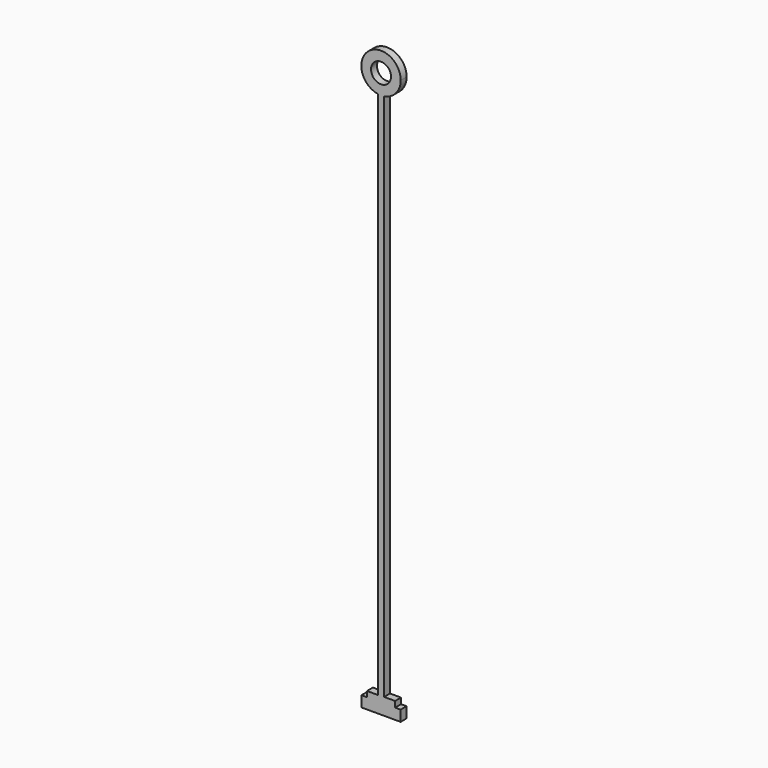
from build123d import *

# Parameters (mm, degrees)
F1_R     = 3.429
F2_DEPTH = 2.54
F3_DEPTH = 25.4


# Not quite as in the source:
# - a feature names something its author has since deleted; it is built from what else it names


with BuildPart() as f2:
    # F1 (on offset) → F2 (new body)
    with BuildSketch(Plane.XZ.offset(25.4)):
        with BuildLine():
            Line((-6.7237908952, -152.7482020624), (-6.7237908952, -156.4639806747))
            Line((-6.7237908952, -156.4639806747), (-2.04e-07, -156.4639806747))
            Line((-2.04e-07, -156.4639806747), (6.7237904873, -156.4639806747))
            Line((6.7237904873, -156.4639806747), (6.7237904873, -152.7482020624))
            Line((6.7237904873, -152.7482020624), (4.8364107652, -152.7482020624))
            Line((4.8364107652, -152.7482020624), (4.8364107652, -150.8608219091))
            Line((4.8364107652, -150.8608219091), (4.8364107652, -150.7428611076))
            Line((4.8364107652, -150.7428611076), (1.0616511053, -150.7428611076))
            Line((1.0616511053, -150.7428611076), (1.0616511053, 30.8865145628))
            ThreePointArc((1.0616511053, 30.8865145628), (-2.065e-07, 30.802726532), (-1.0616515132, 30.8865146276))
            Line((-1.0616515132, 30.8865146276), (-1.0616515132, -150.7428611076))
            Line((-1.0616515132, -150.7428611076), (-1.0616515132, -150.8608219091))
            Line((-1.0616515132, -150.8608219091), (-4.8364111731, -150.8608219091))
            Line((-4.8364111731, -150.8608219091), (-4.8364111731, -152.7482020624))
            Line((-4.8364111731, -152.7482020624), (-6.7237908952, -152.7482020624))
        make_face()
        with BuildLine():
            ThreePointArc((6.7678133299, 37.5705398619), (-4.3942142646, 42.7177894445), (-1.0616515132, 30.8865146276))
            ThreePointArc((-1.0616515132, 30.8865146276), (-2.065e-07, 30.802726532), (1.0616511053, 30.8865145628))
            ThreePointArc((1.0616511053, 30.8865145628), (5.1472494485, 33.1763254403), (6.7678133299, 37.5705398619))
        make_face()
        with Locations((0, 37.5705398619)):
            Circle(F1_R, mode=Mode.SUBTRACT)
        with Locations((0, 37.5705398619)):
            Circle(F1_R)
    extrude(amount=-F2_DEPTH)

    # F1 (on offset) → F3 (cut)
    with BuildSketch(Plane.XZ.offset(25.4)):
        with Locations((0, 37.5705398619)):
            Circle(F1_R)
    extrude(amount=-F3_DEPTH, mode=Mode.SUBTRACT)


solid = f2.part
